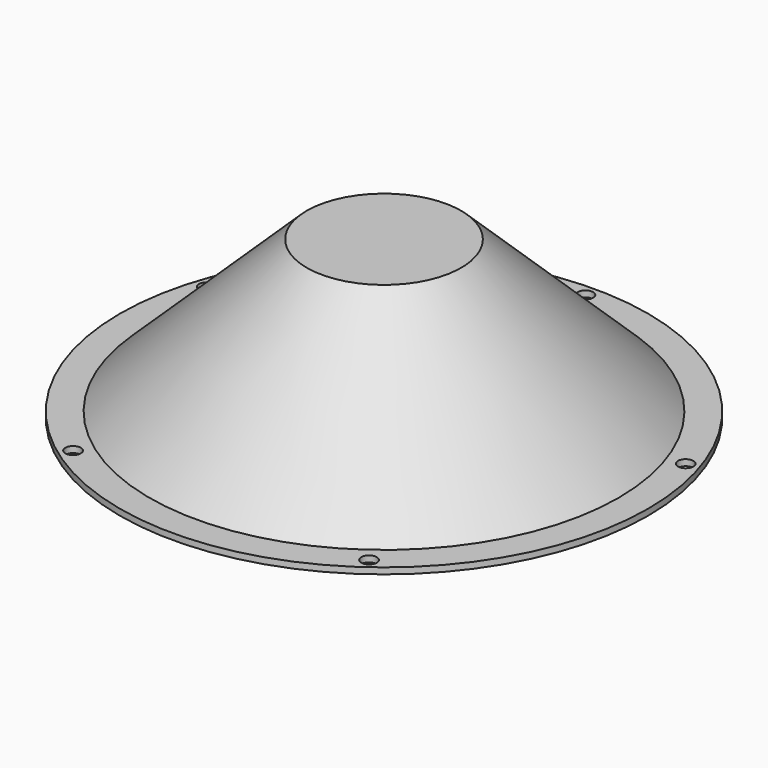
from build123d import *

# Parameters (mm, degrees)
F0_R     = 171
F0_R_2   = 148
F1_DEPTH = 4
F2_R     = 5
F3_DEPTH = 4.001
F4_R     = 151
F4_R_2   = 148
F5_DEPTH = 10


with BuildPart() as f1:
    # F0 (on Top) → F1 (new body)
    with BuildSketch(Plane.XY):
        Circle(F0_R)
        Circle(F0_R_2, mode=Mode.SUBTRACT)
    extrude(amount=F1_DEPTH)

    # F2 (on face) → F3 (cut, through all)
    with BuildSketch(Plane.XY.offset(4)):
        with Locations((0, 163)):
            Circle(F2_R)
        with Locations((-155.0222121561, 50.3697700831)):
            Circle(F2_R)
        with Locations((155.0222121561, 50.3697700831)):
            Circle(F2_R)
        with Locations((95.8089961237, -131.8697700831)):
            Circle(F2_R)
        with Locations((-95.8089961237, -131.8697700831)):
            Circle(F2_R)
    extrude(amount=-F3_DEPTH, mode=Mode.SUBTRACT)

    # F4 (on face) → F5 (join)
    with BuildSketch(Plane(origin=(0, 0, 0), x_dir=(1, 0, 0), z_dir=(0, 0, -1))):
        Circle(F4_R)
        Circle(F4_R_2, mode=Mode.SUBTRACT)
    extrude(amount=F5_DEPTH)

    # F7 (on offset) → F8 (revolve)
    with BuildSketch(Plane.XZ):
        Polygon((-50, 102), (-151.8850358972, 4), (-149, 4), (-49.1942505497, 100), (0, 100), (0, 102), align=None)
    revolve(axis=Axis((0, 0, 51), (0, 0, 1)))


solid = f1.part
